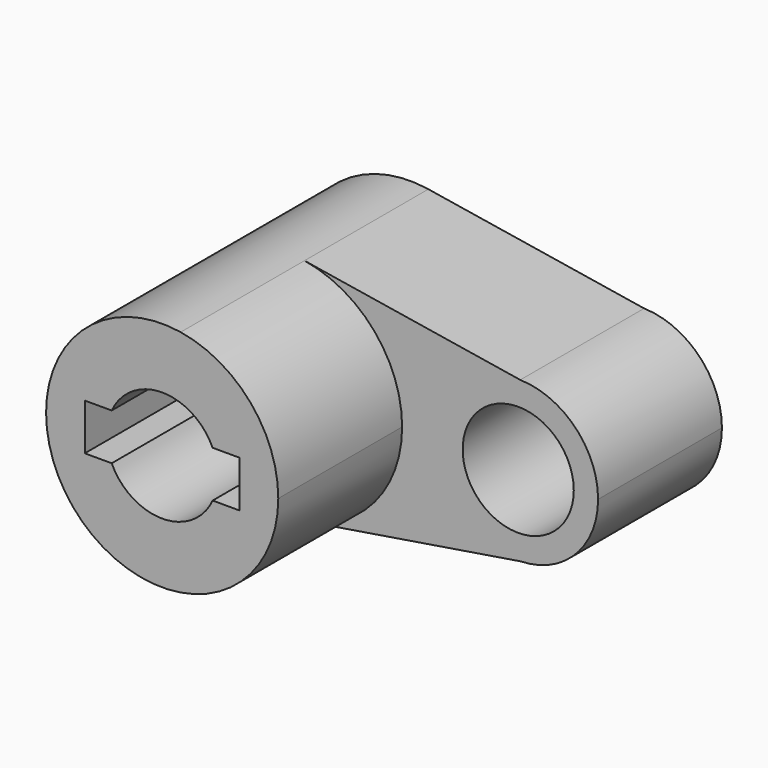
from build123d import *

# Parameters (mm, degrees)
F0_R     = 10.7663
F1_DEPTH = 30
F2_DEPTH = 60


# Not quite as in the source:
# - ends of sketch curves that miss each other by under 0.0002 mm in the source are joined


with BuildPart() as f1:
    # F0 (on Front) → F1 (new body)
    with BuildSketch(Plane.XZ):
        with BuildLine():
            ThreePointArc((3.5818546953, 22.2130663561), (17.1295319645, 14.5886645954), (22.5, 0))
            ThreePointArc((22.5, 0), (17.1295319492, -14.5886646134), (3.5818546487, -22.2130663636))
            Line((3.5818546487, -22.2130663636), (45.4461782926, -15.469383066))
            ThreePointArc((45.4461782926, -15.469383066), (29.5242054073, -0.0258695995), (45.3944581798, 15.4707882881))
            Line((45.3944581798, 15.4707882881), (3.5818546953, 22.2130663561))
        make_face()
        with BuildLine():
            ThreePointArc((60.4758162147, 0), (56.0816390892, 10.8026923778), (45.3944581798, 15.4707882881))
            ThreePointArc((45.3944581798, 15.4707882881), (29.5242054073, -0.0258695995), (45.4461782926, -15.469383066))
            ThreePointArc((45.4461782926, -15.469383066), (56.0996815443, -10.7841530557), (60.4758162147, 0))
        make_face()
        with Locations((45, 0)):
            Circle(F0_R, mode=Mode.SUBTRACT)
    extrude(amount=F1_DEPTH)

    # F0 (on Front) → F2 (join)
    with BuildSketch(Plane.XZ):
        with BuildLine():
            ThreePointArc((3.5818546487, -22.2130663636), (17.1295319492, -14.5886646134), (22.5, 0))
            ThreePointArc((22.5, 0), (17.1295319645, 14.5886645954), (3.5818546953, 22.2130663561))
            ThreePointArc((3.5818546953, 22.2130663561), (-22.5, 2.36e-08), (3.5818546487, -22.2130663636))
        make_face()
        with BuildLine():
            ThreePointArc((-9.780757419, 4.5), (0, 10.7663), (9.780757419, 4.5))
            Line((9.780757419, 4.5), (15, 4.5))
            Line((15, 4.5), (15, -4.5))
            Line((15, -4.5), (9.780757419, -4.5))
            ThreePointArc((9.780757419, -4.5), (0, -10.7663), (-9.780757419, -4.5))
            Line((-9.780757419, -4.5), (-15, -4.5))
            Line((-15, -4.5), (-15, 4.5))
            Line((-15, 4.5), (-9.780757419, 4.5))
        make_face(mode=Mode.SUBTRACT)
    extrude(amount=F2_DEPTH)


solid = f1.part
